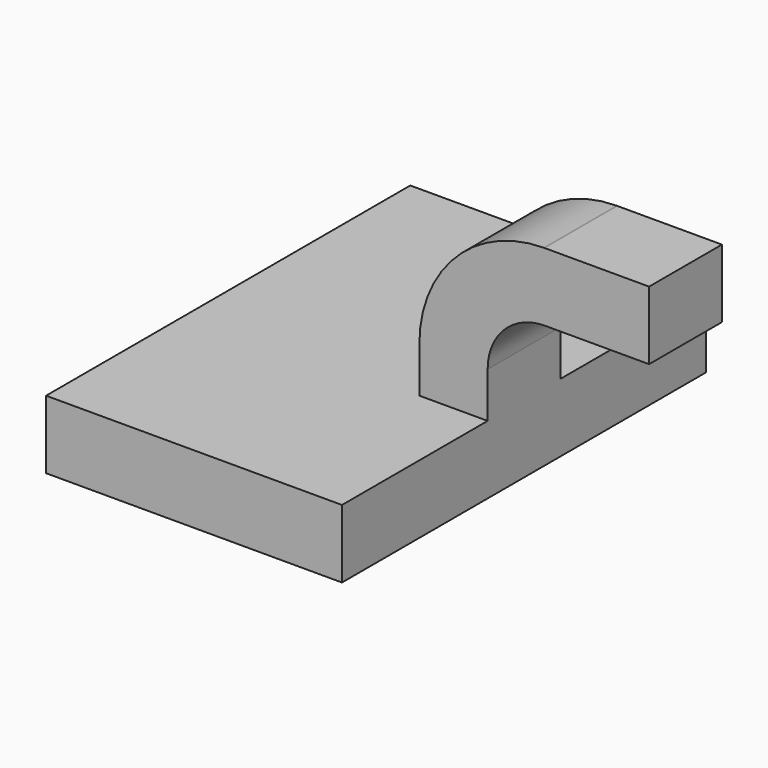
from build123d import *

# Parameters (mm, degrees)
F1_DEPTH = 63.5
F0_W     = 25.0981404377
F0_H     = 19.05
F2_DEPTH = 12.7


# Not quite as in the source:
# - a feature of the source that left no trace in its solid (it failed there, or was rolled back) is left out


with BuildPart() as f1:
    # F0 (on Front) → F1 (new body, symmetric)
    with BuildSketch(Plane.XZ):
        Polygon((-41.275, 9.525), (-41.275, -9.525), (41.275, -9.525), (41.275, 9.525), (22.225, 9.525), align=None)
    extrude(amount=F1_DEPTH, both=True)

    # F0 (on Front) → F2 (join, symmetric)
    with BuildSketch(Plane.XZ):
        with BuildLine():
            Line((22.225, 9.525), (41.275, 9.525))
            Line((41.275, 9.525), (41.275, 22.225))
            ThreePointArc((41.275, 22.225), (45.9246798487, 33.4503201513), (57.15, 38.1))
            Line((57.15, 38.1), (61.2148200089, 38.1))
            Line((61.2148200089, 38.1), (61.2148200089, 57.15))
            Line((61.2148200089, 57.15), (57.15, 57.15))
            add(Edge.make_bspline(
                [(56.9224584332, 57.1492587586), (56.9983070138, 57.1495642251), (57.0741542652, 57.1498113371), (57.15, 57.15)],
                knots=[109.1715172756, 109.1715172756, 109.1715172756, 109.1715172756, 109.3417635215, 109.3417635215, 109.3417635215, 109.3417635215], degree=3))
            ThreePointArc((56.9224584332, 57.1492587586), (32.3739781823, 46.8401247791), (22.225, 22.225))
            Line((22.225, 22.225), (22.225, 9.525))
        make_face()
        with Locations((73.7638902278, 47.625)):
            Rectangle(F0_W, F0_H)
    extrude(amount=F2_DEPTH, both=True)


solid = f1.part
